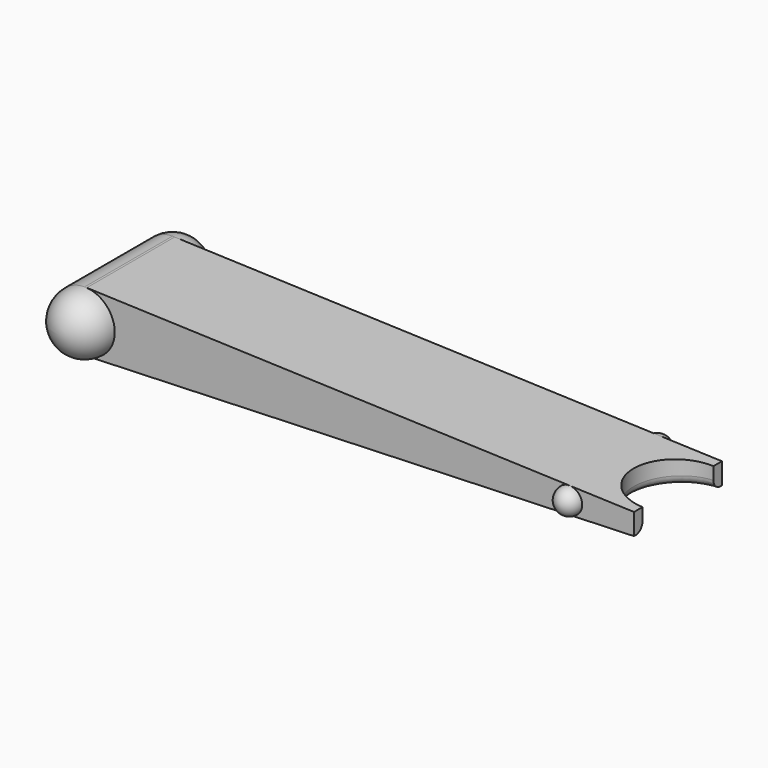
from build123d import *

# Parameters (mm, degrees)
F4_DEPTH = 3.1
F5_DEPTH = 0.5
F6_R     = 0.25


# Not quite as in the source:
# - a feature names something its author has since deleted; it is built from what else it names


with BuildPart() as f1:
    # F0 (on Top) → F1 (revolve)
    with BuildSketch(Plane.XY):
        with BuildLine():
            Line((-14.52249, 3.1), (-13.67249, 3.1))
            Line((-13.67249, 3.1), (-13.67249, 3.95))
            ThreePointArc((-13.67249, 3.95), (-14.273530764, 3.701040764), (-14.52249, 3.1))
        make_face()
    revolve(axis=Axis((-13.67249, 1.55, 0), (0, -1, 0)))



with BuildPart() as f1b:
    # F0 (on Top) → F1, piece 2 (revolve)
    with BuildSketch(Plane.XY):
        with BuildLine():
            Line((-13.67249, -0.85), (-13.67249, 0))
            Line((-13.67249, 0), (-14.52249, 0))
            ThreePointArc((-14.52249, 0), (-14.273530764, -0.601040764), (-13.67249, -0.85))
        make_face()
    revolve(axis=Axis((-13.67249, 1.55, 0), (0, -1, 0)))


with BuildPart() as f2:
    # F0 (on Top) → F2 (revolve)
    with BuildSketch(Plane.XY):
        with BuildLine():
            Line((-0.365, 3.1), (0, 3.1))
            Line((0, 3.1), (0, 3.465))
            ThreePointArc((0, 3.465), (-0.2580939751, 3.3580939751), (-0.365, 3.1))
        make_face()
    revolve(axis=Axis((0, 1.55, 0), (0, 1, 0)))


with BuildPart() as f2b:
    # F0 (on Top) → F2, piece 2 (revolve)
    with BuildSketch(Plane.XY):
        with BuildLine():
            Line((0, -0.365), (0, 0))
            Line((0, 0), (-0.365, 0))
            ThreePointArc((-0.365, 0), (-0.2580939751, -0.2580939751), (0, -0.365))
        make_face()
    revolve(axis=Axis((0, 1.55, 0), (0, 1, 0)))


with BuildPart() as f1_1:
    add(f1.part)

    add(f1b.part)  # F4 merges F1b

    add(f2.part)  # F4 merges F2

    add(f2b.part)  # F4 merges F2b
    # F3 (on face) → F4 (join, through all)
    with BuildSketch(Plane(origin=(0, 0, 0), x_dir=(-1, 0, 0), z_dir=(0, 1, 0))):
        with BuildLine():
            Line((-1.82751, 0), (12.82249, 0))
            ThreePointArc((12.82249, 0), (13.0505296028, 0.579366261), (13.612290622, 0.847865576))
            Line((13.612290622, 0.847865576), (-1.82751, 0.3004333129))
            Line((-1.82751, 0.3004333129), (-1.82751, 0))
        make_face()
        with BuildLine():
            Line((-1.82751, -0.3004333129), (13.612290622, -0.847865576))
            ThreePointArc((13.612290622, -0.847865576), (13.0505296028, -0.579366261), (12.82249, 0))
            Line((12.82249, 0), (-1.82751, 0))
            Line((-1.82751, 0), (-1.82751, -0.3004333129))
        make_face()
        with BuildLine():
            Line((12.82249, 0), (14.52249, 0))
            ThreePointArc((14.52249, 0), (14.273530764, 0.601040764), (13.67249, 0.85))
            Line((13.67249, 0.85), (13.612290622, 0.847865576))
            ThreePointArc((13.612290622, 0.847865576), (13.0505296028, 0.579366261), (12.82249, 0))
        make_face()
        with BuildLine():
            Line((13.612290622, -0.847865576), (13.67249, -0.85))
            ThreePointArc((13.67249, -0.85), (14.273530764, -0.601040764), (14.52249, 0))
            Line((14.52249, 0), (12.82249, 0))
            ThreePointArc((12.82249, 0), (13.0505296028, -0.579366261), (13.612290622, -0.847865576))
        make_face()
    extrude(amount=F4_DEPTH)

    # F0 (on Top) → F5 (cut, symmetric)
    with BuildSketch(Plane.XY):
        with BuildLine():
            ThreePointArc((1.82751, 2.8), (0.57751, 1.55), (1.82751, 0.3))
            Line((1.82751, 0.3), (1.82751, 2.8))
        make_face()
    extrude(amount=F5_DEPTH, both=True, mode=Mode.SUBTRACT)

    # F6
    f6_edges = [f1_1.edges().sort_by_distance(p)[0] for p in [
        (0.57751, 1.55, -0.344753),
    ]]
    fillet(f6_edges, radius=F6_R)


solid = f1_1.part
